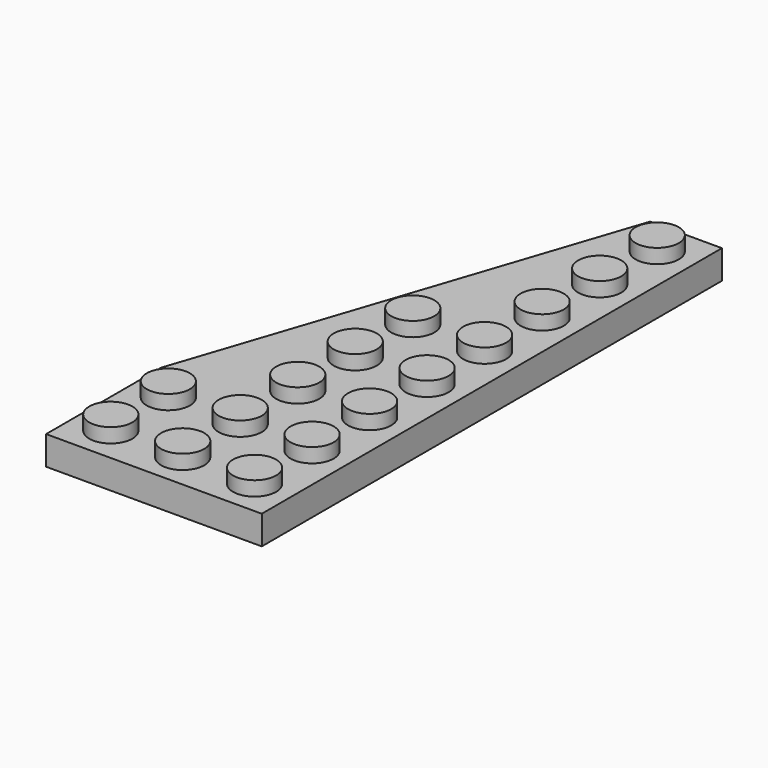
from build123d import *

# Parameters (mm, degrees)
F0_R     = 2.38125
F1_DEPTH = 3.175
F2_DEPTH = 4.7625
F3_T     = -1.5875
F4_R     = 3.175
F4_R_2   = 2.38125
F5_DEPTH = 1.5875


with BuildPart() as f1:
    # F0 (on Top) → F1 (new body)
    with BuildSketch(Plane.XY):
        Polygon((11.90625, 31.75), (3.96875, 31.75), (-11.90625, -15.875), (-11.90625, -31.75), (11.90625, -31.75), align=None)
        with Locations((-7.9375, -27.78125)):
            Circle(F0_R, mode=Mode.SUBTRACT)
        with Locations((-7.9375, -19.84375)):
            Circle(F0_R, mode=Mode.SUBTRACT)
        with Locations((0, -27.78125)):
            Circle(F0_R, mode=Mode.SUBTRACT)
        with Locations((0, -19.84375)):
            Circle(F0_R, mode=Mode.SUBTRACT)
        with Locations((7.9375, -27.78125)):
            Circle(F0_R, mode=Mode.SUBTRACT)
        with Locations((7.9375, -19.84375)):
            Circle(F0_R, mode=Mode.SUBTRACT)
        with Locations((0, -11.90625)):
            Circle(F0_R, mode=Mode.SUBTRACT)
        with Locations((0, -3.96875)):
            Circle(F0_R, mode=Mode.SUBTRACT)
        with Locations((7.9375, -11.90625)):
            Circle(F0_R, mode=Mode.SUBTRACT)
        with Locations((7.9375, -3.96875)):
            Circle(F0_R, mode=Mode.SUBTRACT)
        with Locations((0, 3.96875)):
            Circle(F0_R, mode=Mode.SUBTRACT)
        with Locations((7.9375, 3.96875)):
            Circle(F0_R, mode=Mode.SUBTRACT)
        with Locations((7.9375, 11.90625)):
            Circle(F0_R, mode=Mode.SUBTRACT)
        with Locations((7.9375, 19.84375)):
            Circle(F0_R, mode=Mode.SUBTRACT)
        with Locations((7.9375, 27.78125)):
            Circle(F0_R, mode=Mode.SUBTRACT)
    extrude(amount=F1_DEPTH)

    # F0 (on Top) → F2 (join)
    with BuildSketch(Plane.XY):
        with Locations((7.9375, 27.78125)):
            Circle(F0_R)
        with Locations((7.9375, 19.84375)):
            Circle(F0_R)
        with Locations((7.9375, 11.90625)):
            Circle(F0_R)
        with Locations((0, 3.96875)):
            Circle(F0_R)
        with Locations((7.9375, 3.96875)):
            Circle(F0_R)
        with Locations((7.9375, -3.96875)):
            Circle(F0_R)
        with Locations((0, -3.96875)):
            Circle(F0_R)
        with Locations((0, -11.90625)):
            Circle(F0_R)
        with Locations((7.9375, -11.90625)):
            Circle(F0_R)
        with Locations((7.9375, -19.84375)):
            Circle(F0_R)
        with Locations((0, -19.84375)):
            Circle(F0_R)
        with Locations((-7.9375, -19.84375)):
            Circle(F0_R)
        with Locations((-7.9375, -27.78125)):
            Circle(F0_R)
        with Locations((0, -27.78125)):
            Circle(F0_R)
        with Locations((7.9375, -27.78125)):
            Circle(F0_R)
    extrude(amount=F2_DEPTH)

    # F3
    f3_openings = [f1.faces().sort_by_distance(p)[0] for p in [
        (2.204861, -5.291667, 0),
    ]]
    offset(amount=F3_T, openings=f3_openings, kind=Kind.INTERSECTION)

    # F4 (on face) → F5 (join)
    with BuildSketch(Plane(origin=(0, 0, 1.5875), x_dir=(1, 0, 0), z_dir=(0, 0, -1))):
        with BuildLine():
            ThreePointArc((-0.79375, 23.8125), (-2.7537301022, 26.7458175157), (-6.2138140303, 26.0575640303))
            Line((-6.2138140303, 26.0575640303), (-5.6525480227, 25.4962980227))
            ThreePointArc((-5.6525480227, 25.4962980227), (-3.0574850767, 26.0124881368), (-1.5875, 23.8125))
            ThreePointArc((-1.5875, 23.8125), (-1.7687618632, 22.9012350767), (-2.2849519773, 22.1287019773))
            Line((-2.2849519773, 22.1287019773), (-1.7236859697, 21.5674359697))
            ThreePointArc((-1.7236859697, 21.5674359697), (-1.0354324843, 22.5974801022), (-0.79375, 23.8125))
        make_face()
        with BuildLine():
            Line((-5.6525480227, 25.4962980227), (-6.2138140303, 26.0575640303))
            ThreePointArc((-6.2138140303, 26.0575640303), (-6.2138140303, 21.5674359697), (-1.7236859697, 21.5674359697))
            Line((-1.7236859697, 21.5674359697), (-2.2849519773, 22.1287019773))
            ThreePointArc((-2.2849519773, 22.1287019773), (-5.6525480227, 22.1287019773), (-5.6525480227, 25.4962980227))
        make_face()
        with Locations((-3.96875, 15.875)):
            Circle(F4_R)
        with Locations((-3.96875, 15.875)):
            Circle(F4_R_2, mode=Mode.SUBTRACT)
        with Locations((-3.96875, 7.9375)):
            Circle(F4_R)
        with Locations((-3.96875, 7.9375)):
            Circle(F4_R_2, mode=Mode.SUBTRACT)
        with BuildLine():
            ThreePointArc((-3.8832617755, -3.1738488879), (-1.6936620772, -2.2146331397), (-0.79375, 0))
            ThreePointArc((-0.79375, 0), (-2.5107405764, 2.8204314423), (-5.8046687532, 2.590372045))
            Line((-5.8046687532, 2.590372045), (-5.5381726179, 1.7908836392))
            ThreePointArc((-5.5381726179, 1.7908836392), (-2.9856009895, 2.1688175547), (-1.5875, 0))
            ThreePointArc((-1.5875, 0), (-2.350212624, -1.7466219754), (-4.1497579108, -2.3743604821))
            Line((-4.1497579108, -2.3743604821), (-3.8832617755, -3.1738488879))
        make_face()
        with BuildLine():
            ThreePointArc((7.14375, -23.8125), (5.4267594236, -20.9920685577), (2.1328312468, -21.222127955))
            Line((2.1328312468, -21.222127955), (2.3993273821, -22.0216163608))
            ThreePointArc((2.3993273821, -22.0216163608), (4.9518990105, -21.6436824453), (6.35, -23.8125))
            ThreePointArc((6.35, -23.8125), (5.587287376, -25.5591219754), (3.7877420892, -26.1868604821))
            Line((3.7877420892, -26.1868604821), (4.0542382245, -26.9863488879))
            ThreePointArc((4.0542382245, -26.9863488879), (6.2438379228, -26.0271331397), (7.14375, -23.8125))
        make_face()
        with Locations((3.96875, 23.8125)):
            Circle(F4_R)
        with Locations((3.96875, 23.8125)):
            Circle(F4_R_2, mode=Mode.SUBTRACT)
        with Locations((3.96875, 15.875)):
            Circle(F4_R)
        with Locations((3.96875, 15.875)):
            Circle(F4_R_2, mode=Mode.SUBTRACT)
        with Locations((3.96875, 7.9375)):
            Circle(F4_R)
        with Locations((3.96875, 7.9375)):
            Circle(F4_R_2, mode=Mode.SUBTRACT)
        with Locations((3.96875, 0)):
            Circle(F4_R)
        with Locations((3.96875, 0)):
            Circle(F4_R_2, mode=Mode.SUBTRACT)
        with Locations((3.96875, -7.9375)):
            Circle(F4_R)
        with Locations((3.96875, -7.9375)):
            Circle(F4_R_2, mode=Mode.SUBTRACT)
        with Locations((3.96875, -15.875)):
            Circle(F4_R)
        with Locations((3.96875, -15.875)):
            Circle(F4_R_2, mode=Mode.SUBTRACT)
    extrude(amount=F5_DEPTH)


solid = f1.part
